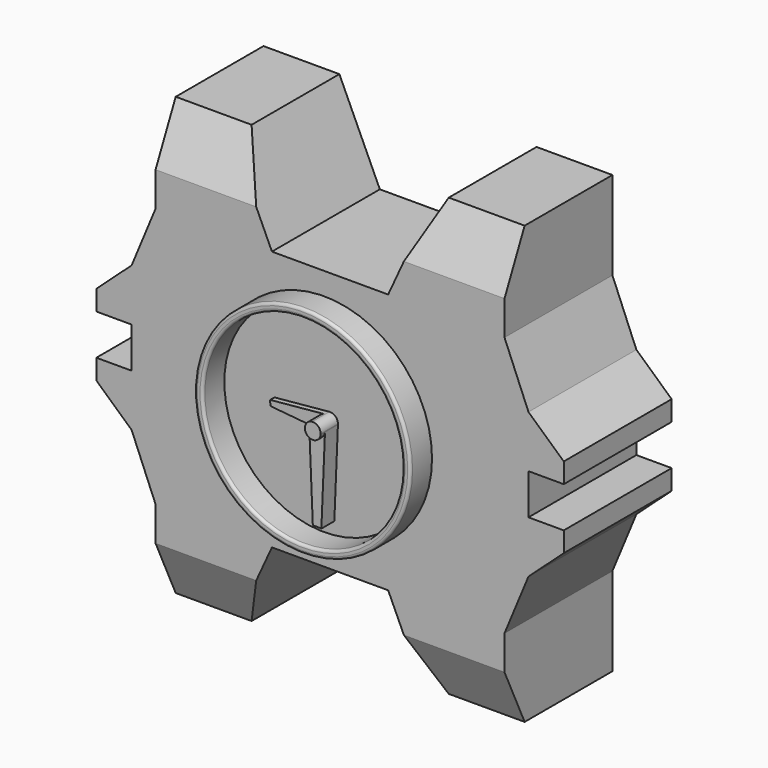
from build123d import *

# Parameters (mm, degrees)
F1_DEPTH = 25
F2_SIZE2 = 4.6630765815
F2_SIZE  = 10
F3_R     = 20
F3_R_2   = 18.5
F4_DEPTH = 5
F5_R     = 0.5
F7_DEPTH = 3
F8_DEPTH = 4
F9_DEPTH = 1


with BuildPart() as f1:
    # F0 (on Front) → F1 (new body)
    with BuildSketch(Plane.XZ):
        Polygon((-10.7714766636, 24.1296291351), (-32.3379188776, 24.1296291351), (-32.3379188776, -24.1296291351), (-10.7714766636, -24.1296291351), (10.7714766636, -24.1296291351), (32.3379188776, -24.1296291351), (32.3379188776, 24.1296291351), (10.7714766636, 24.1296291351), align=None)
        Polygon((-10.7714766636, -24.1296291351), (-32.3379188776, -24.1296291351), (-32.3379188776, -40.4889471829), (-18.2706620544, -40.4889471829), align=None)
        Polygon((32.3379188776, -24.1296291351), (10.7714766636, -24.1296291351), (18.2706620544, -40.4889471829), (32.3379188776, -40.4889471829), align=None)
        Polygon((36.7772430182, 13.4279271588), (32.3379188776, 24.1296291351), (32.3379188776, -24.1296291351), (36.7772430182, -13.4279271588), (43.317168951, -7.4825375341), (43.317168951, -3.7666687276), (36.7772430182, -3.7666687276), (36.7772430182, 3.7666687276), (43.317168951, 3.7666687276), (43.317168951, 7.4825375341), align=None)
        Polygon((18.2706620544, 40.4889471829), (10.7714766636, 24.1296291351), (32.3379188776, 24.1296291351), (32.3379188776, 40.4889471829), align=None)
        Polygon((-32.3379188776, 40.4889471829), (-32.3379188776, 24.1296291351), (-10.7714766636, 24.1296291351), (-18.2706620544, 40.4889471829), align=None)
        Polygon((-32.3379188776, -24.1296291351), (-32.3379188776, 24.1296291351), (-36.7772430182, 13.4279271588), (-43.317168951, 7.4825375341), (-43.317168951, 3.7666687276), (-36.7772430182, 3.7666687276), (-36.7772430182, -3.7666687276), (-43.317168951, -3.7666687276), (-43.317168951, -7.4825375341), (-36.7772430182, -13.4279271588), align=None)
    extrude(amount=F1_DEPTH)

    # F2
    f2_edges = [f1.edges().sort_by_distance(p)[0] for p in [
        (-25.30429, -25, -40.488947),
        (25.30429, -25, -40.488947),
        (25.30429, -25, 40.488947),
        (-25.30429, -25, 40.488947),
    ]]
    f2_side = f1.faces().sort_by_distance((0, -25, 0))[0]
    chamfer(f2_edges, length=F2_SIZE, length2=F2_SIZE2, reference=f2_side)

    # F3 (on face) → F4 (join)
    with BuildSketch(Plane.XZ.offset(25)):
        with Locations((-1.1007853685, 0)):
            Circle(F3_R)
        with Locations((-1.1007853685, 0)):
            Circle(F3_R_2, mode=Mode.SUBTRACT)
    extrude(amount=F4_DEPTH)

    # F5
    f5_edges = [f1.edges().sort_by_distance(p)[0] for p in [
        (-21.100785, -30, 0),
        (-19.600785, -30, 0),
    ]]
    fillet(f5_edges, radius=F5_R)

    # F6 (on face) → F7 (join)
    with BuildSketch(Plane.XZ.offset(25)):
        with BuildLine():
            Line((0.7930111024, -16.0924680531), (1.4582137539, -0.1216838649))
            ThreePointArc((1.4582137539, -0.1216838649), (0.9907412633, -1.0768593521), (0, -1.4632820354))
            ThreePointArc((0, -1.4632820354), (-0.1366349733, -1.4568888767), (-0.2720760154, -1.4377652649))
            Line((-0.2720760154, -1.4377652649), (-1.407833944, -1.3312477008))
            Line((-1.407833944, -1.3312477008), (-0.7930111024, -16.0924680531))
            Line((-0.7930111024, -16.0924680531), (0, -16.0594381729))
            Line((0, -16.0594381729), (0.7930111024, -16.0924680531))
        make_face()
        with BuildLine():
            ThreePointArc((-0.2720760154, -1.4377652649), (-0.1366349733, -1.4568888767), (0, -1.4632820354))
            Line((0, -1.4632820354), (-0.2720760154, -1.4377652649))
        make_face()
        with BuildLine():
            ThreePointArc((-0.2720760154, -1.4377652649), (-1.0869651486, -0.9796433436), (-1.4582137539, -0.1216838649))
            Line((-1.4582137539, -0.1216838649), (-1.407833944, -1.3312477008))
            Line((-1.407833944, -1.3312477008), (-0.2720760154, -1.4377652649))
        make_face()
    extrude(amount=F7_DEPTH)

    # F6 (on face) → F8 (join)
    with BuildSketch(Plane.XZ.offset(25)):
        with BuildLine():
            Line((1.4582137539, -0.1216838649), (1.4632820354, 0))
            ThreePointArc((1.4632820354, 0), (0.9847877966, 1.0823064772), (-0.1377590249, 1.4567830195))
            ThreePointArc((-0.1377590249, 1.4567830195), (-1.0823064772, 0.9847877966), (-1.4632820354, 0))
            Line((-1.4632820354, 0), (-1.4582137539, -0.1216838649))
            ThreePointArc((-1.4582137539, -0.1216838649), (-1.0869651486, -0.9796433436), (-0.2720760154, -1.4377652649))
            Line((-0.2720760154, -1.4377652649), (0, -1.4632820354))
            ThreePointArc((0, -1.4632820354), (0.9907412633, -1.0768593521), (1.4582137539, -0.1216838649))
        make_face()
    extrude(amount=F8_DEPTH)


with BuildPart() as f9:
    # F6 (on face) → F9 (new body)
    with BuildSketch(Plane.XZ.offset(25)):
        with BuildLine():
            ThreePointArc((-1.4632820354, 0), (-1.0823064772, 0.9847877966), (-0.1377590249, 1.4567830195))
            Line((-0.1377590249, 1.4567830195), (-10.3039735789, 0.4954265713))
            Line((-10.3039735789, 0.4954265713), (-10.2833384576, 0))
            Line((-10.2833384576, 0), (-10.2624790743, -0.5008108565))
            Line((-10.2624790743, -0.5008108565), (-1.407833944, -1.3312477008))
            Line((-1.407833944, -1.3312477008), (-1.4582137539, -0.1216838649))
            ThreePointArc((-1.4582137539, -0.1216838649), (-1.4620144159, -0.0608946846), (-1.4632820354, 0))
        make_face()
        with BuildLine():
            ThreePointArc((-0.2720760154, -1.4377652649), (-1.0869651486, -0.9796433436), (-1.4582137539, -0.1216838649))
            Line((-1.4582137539, -0.1216838649), (-1.407833944, -1.3312477008))
            Line((-1.407833944, -1.3312477008), (-0.2720760154, -1.4377652649))
        make_face()
    extrude(amount=F9_DEPTH)


solid = Compound([f1.part, f9.part])
